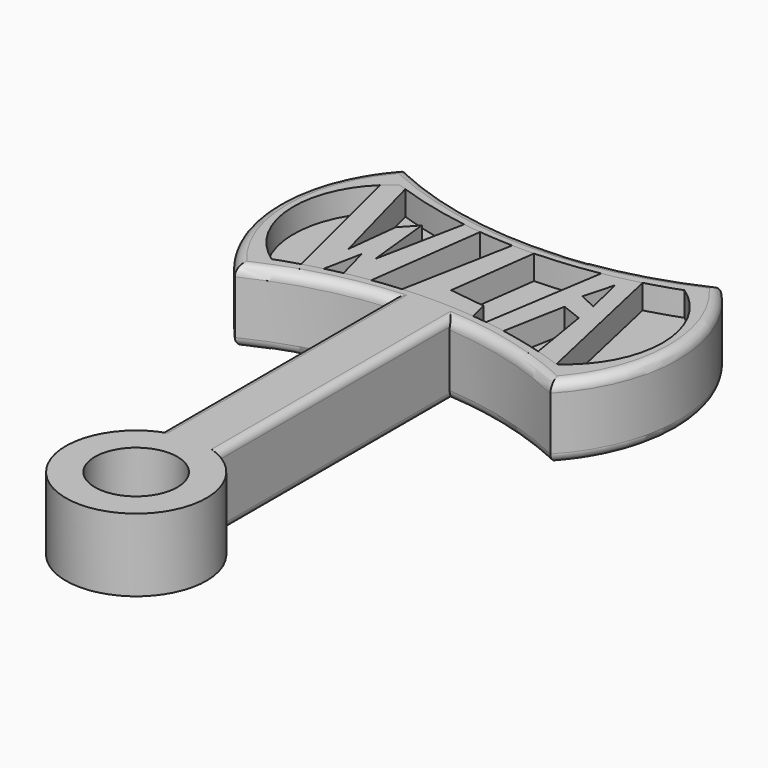
from build123d import *
from build123d import SkipClean  # not in build123d's __all__

# Parameters (mm, degrees)
F0_R     = 8.5
F1_DEPTH = 15
F2_R     = 1.5
F4_R     = 2
F5_DEPTH = 5
F7_DEPTH = 5


with BuildPart() as f1:
    # F0 (on Top) → F1 (new body)
    with BuildSketch(Plane.XY):
        with BuildLine():
            Line((-32.5, -22), (-32.5, 22))
            ThreePointArc((-32.5, 22), (-41.2620999228, 0), (-32.5, -22))
        make_face()
        with BuildLine():
            ThreePointArc((32.5, 22), (0, 14.592529173), (-32.5, 22))
            Line((-32.5, 22), (0, 0))
            Line((0, 0), (32.5, 22))
        make_face()
        Polygon((0, 0), (-32.5, 22), (-32.5, -22), align=None)
        with BuildLine():
            Line((0, 0), (-32.5, -22))
            ThreePointArc((-32.5, -22), (-19.5807119119, -17.1936637052), (-6, -14.8329144067))
            ThreePointArc((-6, -14.8329144067), (0, -14.592529173), (6, -14.8329144067))
            ThreePointArc((6, -14.8329144067), (19.5807119119, -17.1936637052), (32.5, -22))
            Line((32.5, -22), (0, 0))
        make_face()
        Polygon((32.5, -22), (32.5, 22), (0, 0), align=None)
        with BuildLine():
            ThreePointArc((32.5, -22), (41.2620999228, 0), (32.5, 22))
            Line((32.5, 22), (32.5, -22))
        make_face()
        with BuildLine():
            ThreePointArc((6, -14.8329144067), (0, -14.592529173), (-6, -14.8329144067))
            Line((-6, -14.8329144067), (-6, -74.8329144067))
            Line((-6, -74.8329144067), (6, -74.8329144067))
            Line((6, -74.8329144067), (6, -14.8329144067))
        make_face()
        with BuildLine():
            Line((6, -74.8329144067), (-6, -74.8329144067))
            ThreePointArc((-6, -74.8329144067), (0, -102.5332931892), (6, -74.8329144067))
        make_face()
        with Locations((0, -88.0332931892)):
            Circle(F0_R, mode=Mode.SUBTRACT)
    extrude(amount=F1_DEPTH)

    # F2
    f2_edges = [f1.edges().sort_by_distance(p)[0] for p in [
        (-6, -44.832914, 15),
        (6, -44.832914, 15),
        (6, -44.832914, 0),
        (-6, -44.832914, 0),
    ]]
    fillet(f2_edges, radius=F2_R)

    # F4
    f4_edges = [f1.edges().sort_by_distance(p)[0] for p in [
        (-19.580712, -17.193664, 15),
        (-41.2621, 0, 15),
        (19.580712, -17.193664, 15),
        (-19.580712, -17.193664, 0),
        (-41.2621, 0, 0),
        (0, 14.592529, 0),
        (41.2621, 0, 0),
        (19.580712, -17.193664, 0),
        (41.2621, 0, 15),
        (0, 14.592529, 15),
    ]]
    fillet(f4_edges, radius=F4_R)

    # F3 (on face) → F5 (cut)
    with BuildSketch(Plane.XY.offset(15)):
        with BuildLine():
            Line((-29.3147544782, -16.5), (-29.3147544782, 16.5))
            ThreePointArc((-29.3147544782, 16.5), (-38.0120999228, 0), (-29.3147544782, -16.5))
        make_face()
        with BuildLine():
            ThreePointArc((0, 11.342529173), (-14.8824925286, 12.6417227993), (-29.3147544782, 16.5))
            Line((-29.3147544782, 16.5), (0, 0))
            Line((0, 0), (0, 11.342529173))
        make_face()
        Polygon((0, 0), (-29.3147544782, 16.5), (-29.3147544782, -16.5), align=None)
        with BuildLine():
            Line((0, 0), (-29.3147544782, -16.5))
            ThreePointArc((-29.3147544782, -16.5), (-14.8824925285, -12.6417227993), (0, -11.342529173))
            Line((0, -11.342529173), (0, 0))
        make_face()
        with BuildLine():
            ThreePointArc((29.3147544782, 16.5), (14.8824925286, 12.6417227993), (0, 11.342529173))
            Line((0, 11.342529173), (0, 0))
            Line((0, 0), (29.3147544782, 16.5))
        make_face()
        Polygon((29.3147544782, 16.5), (0, 0), (29.3147544782, -16.5), align=None)
        with BuildLine():
            Line((29.3147544782, -16.5), (0, 0))
            Line((0, 0), (0, -11.342529173))
            ThreePointArc((0, -11.342529173), (14.8824925286, -12.6417227993), (29.3147544782, -16.5))
        make_face()
        with BuildLine():
            ThreePointArc((29.3147544782, -16.5), (38.0120999228, 0), (29.3147544782, 16.5))
            Line((29.3147544782, 16.5), (29.3147544782, -16.5))
        make_face()
    with SkipClean():  # cleaning this boolean's faces spoils the solid; the shape is the same uncleaned
        extrude(amount=-F5_DEPTH, mode=Mode.SUBTRACT)

    # F6 (on face) → F7 (join)
    with BuildSketch(Plane.XY.offset(10)):
        with BuildLine():
            Line((15.2079802839, 12.699633284), (11.3304843403, -12.0931563405))
            ThreePointArc((11.3304843403, -12.0931563405), (13.3952654965, -12.3935064492), (15.4521416161, -12.7439233999))
            Line((15.4521416161, -12.7439233999), (17.8190562874, 0))
            Line((17.8190562874, 0), (22.0686495304, -1.6748139169))
            Line((22.0686495304, -1.6748139169), (24.2379181726, -14.8333900519))
            ThreePointArc((24.2379181726, -14.8333900519), (26.7892998078, -15.6272055953), (29.3147544782, -16.5))
            Line((29.3147544782, -16.5), (22.4350078947, 14.3243580948))
            ThreePointArc((22.4350078947, 14.3243580948), (18.8390172894, 13.4340497811), (15.2079802839, 12.699633284))
        make_face()
        Polygon((17.8190562874, 4.6145855449), (19.5188932121, 10.9039852396), (21.3887151331, 2.9147479217), align=None, mode=Mode.SUBTRACT)
        with BuildLine():
            Line((-2.0585943572, 11.3672025947), (-6.3891717286, -11.5804961029))
            ThreePointArc((-6.3891717286, -11.5804961029), (1.0259296068, -11.3486565705), (8.4333769686, -11.7575587165))
            Line((8.4333769686, -11.7575587165), (7.4048662885, -7.905074934))
            Line((7.4048662885, -7.905074934), (0, -6.9299801253))
            Line((0, -6.9299801253), (2.4106339203, 11.3763647448))
            ThreePointArc((2.4106339203, 11.3763647448), (0.1760793848, 11.3427096587), (-2.0585943572, 11.3672025947))
        make_face()
        with BuildLine():
            ThreePointArc((-29.3147544782, 16.5), (-30.604070915, 15.5384126129), (-31.8119491831, 14.4763310404))
            Line((-31.8119491831, 14.4763310404), (-24.5027556892, -14.9117551872))
            ThreePointArc((-24.5027556892, -14.9117551872), (-22.5955271512, -14.3679613691), (-20.6762515008, -13.8683481283))
            Line((-20.6762515008, -13.8683481283), (-19.114445895, -6.066611968))
            Line((-19.114445895, -6.066611968), (-17.2392854565, -13.0903846112))
            ThreePointArc((-17.2392854565, -13.0903846112), (-14.7242186042, -12.614029589), (-12.1960735351, -12.2128340149))
            Line((-12.1960735351, -12.2128340149), (-9.0315309989, 11.8186900319))
            ThreePointArc((-9.0315309989, 11.8186900319), (-10.8625432372, 12.0321900371), (-12.6885517924, 12.2849366013))
            Line((-12.6885517924, 12.2849366013), (-16.3512527943, -6.066611968))
            Line((-16.3512527943, -6.066611968), (-17.7929196507, 7.7493544668))
            Line((-17.7929196507, 7.7493544668), (-20.6762515008, 4.6145855449))
            Line((-20.6762515008, 4.6145855449), (-21.8776389956, -6.066611968))
            Line((-21.8776389956, -6.066611968), (-27.7557073698, 15.9508191787))
            ThreePointArc((-27.7557073698, 15.9508191787), (-28.5365520654, 16.2216590548), (-29.3147544782, 16.5))
        make_face()
    with SkipClean():  # cleaning this boolean's faces spoils the solid; the shape is the same uncleaned
        extrude(amount=F7_DEPTH)


solid = f1.part
